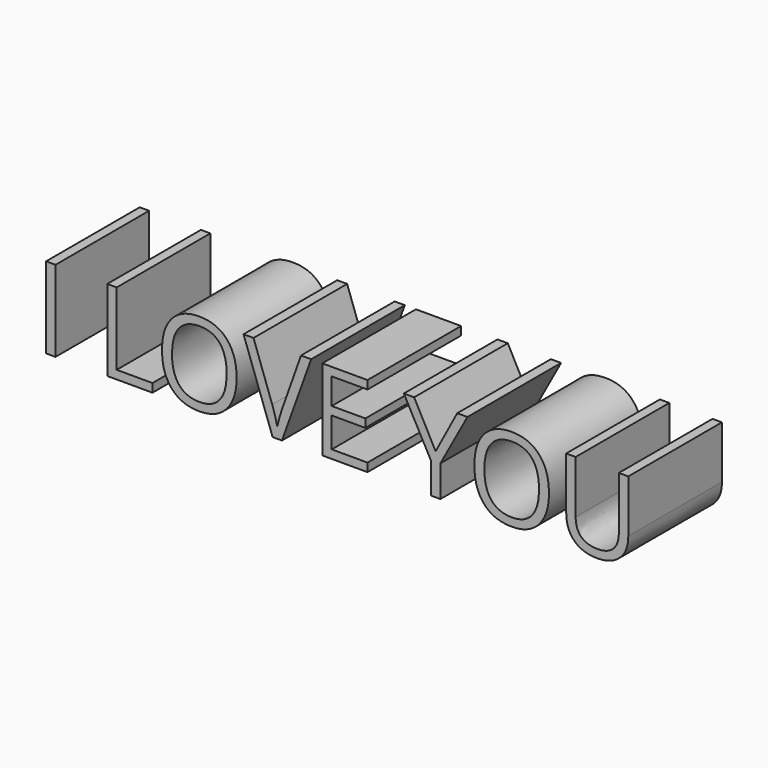
from build123d import *

# Parameters (mm, degrees)
F0_TEXT_SIZE = 24.6530321116
F1_DEPTH     = 25.4


# Not quite as in the source:
# - Text() gives the source's letters only with a copy of the font that has no kerning and outlines rounded to 1/6400 em; it was checked with that copy


with BuildPart() as f1:
    # F0 (on Front) → F1 (new body)
    with BuildSketch(Plane.XZ):
        with Locations((-68.9819902182, 30.8036375791)):
            Text('I LOVE YOU', F0_TEXT_SIZE, font='Open Sans', text_align=(TextAlign.LEFT, TextAlign.BOTTOM))
    extrude(amount=F1_DEPTH)


solid = f1.part
